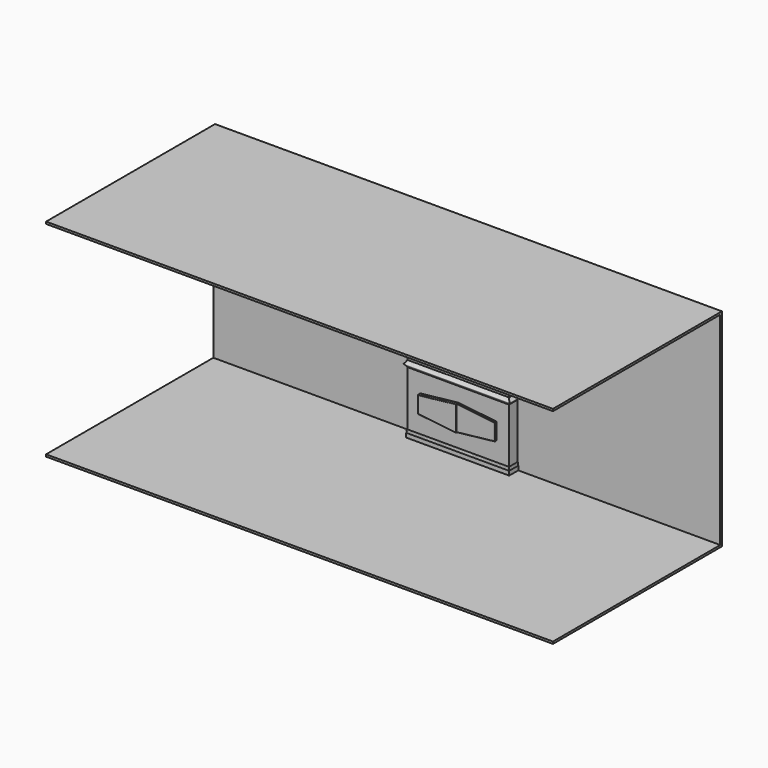
from build123d import *

# Parameters (mm, degrees)
F0_W      = 2438.4
F0_H      = 2438.4
F0_W_2    = 3657.6
F1_DEPTH  = 25.4
F2_W      = 6096
F2_H      = 2540
F3_DEPTH  = 25.4
F4_W      = 6096
F4_H      = 2540
F5_DEPTH  = 25.4
F6_W      = 1219.2
F6_H      = 2133.6
F7_DEPTH  = 127
F8_W      = 762
F8_H      = 762
F9_DEPTH  = 38.1
F15_DEPTH = 190.501
F16_R     = 25.4
F22_DEPTH = 38.1
F23_DEPTH = 25.4
F24_R     = 5.08
F24_2_R   = 5.08
F25_W     = 711.2
F25_H     = 711.2
F26_DEPTH = 6.35


with BuildPart() as f1:
    # F0 (on Front) → F1 (new body)
    with BuildSketch(Plane.XZ):
        with Locations((-1219.2, 1219.2)):
            Rectangle(F0_W, F0_H)
        with Locations((1828.8, 1219.2)):
            Rectangle(F0_W_2, F0_H)
    extrude(amount=-F1_DEPTH)

    # F2 (on face) → F3 (join)
    with BuildSketch(Plane.XY.offset(2438.4)):
        with Locations((609.6, -1244.6)):
            Rectangle(F2_W, F2_H)
    extrude(amount=F3_DEPTH)

    # F4 (on face) → F5 (join)
    with BuildSketch(Plane(origin=(0, 0, 0), x_dir=(1, 0, 0), z_dir=(0, 0, -1))):
        with Locations((609.6, 1244.6)):
            Rectangle(F4_W, F4_H)
    extrude(amount=F5_DEPTH)


with BuildPart() as f7:
    # F6 (on Front) → F7 (new body)
    with BuildSketch(Plane.XZ):
        with Locations((609.6, 1066.8)):
            Rectangle(F6_W, F6_H)
    extrude(amount=F7_DEPTH)


with BuildPart() as f9:
    # F8 (on face) → F9 (new body)
    with BuildSketch(Plane.XZ.offset(127)):
        with Locations((609.6, 1397)):
            Rectangle(F8_W, F8_H)
    extrude(amount=F9_DEPTH)

    # F14 (on face) → F15 (cut, through all)
    with BuildSketch(Plane.XZ.offset(165.1)):
        with BuildLine():
            ThreePointArc((444.5, 1593.85), (442.6401280605, 1598.3401280605), (438.15, 1600.2))
            Line((438.15, 1600.2), (400.05, 1600.2))
            ThreePointArc((400.05, 1600.2), (395.5598719395, 1598.3401280605), (393.7, 1593.85))
            Line((393.7, 1593.85), (393.7, 1200.15))
            ThreePointArc((393.7, 1200.15), (395.5598719395, 1195.6598719395), (400.05, 1193.8))
            Line((400.05, 1193.8), (438.15, 1193.8))
            ThreePointArc((438.15, 1193.8), (442.6401280605, 1195.6598719395), (444.5, 1200.15))
            Line((444.5, 1200.15), (444.5, 1593.85))
        make_face()
        with BuildLine():
            Line((527.05, 1193.8), (565.15, 1193.8))
            ThreePointArc((565.15, 1193.8), (569.6401280605, 1195.6598719395), (571.5, 1200.15))
            Line((571.5, 1200.15), (571.5, 1593.85))
            ThreePointArc((571.5, 1593.85), (569.6401280605, 1598.3401280605), (565.15, 1600.2))
            Line((565.15, 1600.2), (527.05, 1600.2))
            ThreePointArc((527.05, 1600.2), (522.5598719395, 1598.3401280605), (520.7, 1593.85))
            Line((520.7, 1593.85), (520.7, 1200.15))
            ThreePointArc((520.7, 1200.15), (522.5598719395, 1195.6598719395), (527.05, 1193.8))
        make_face()
        with BuildLine():
            Line((654.05, 1193.8), (692.15, 1193.8))
            ThreePointArc((692.15, 1193.8), (696.6401280605, 1195.6598719395), (698.5, 1200.15))
            Line((698.5, 1200.15), (698.5, 1593.85))
            ThreePointArc((698.5, 1593.85), (696.6401280605, 1598.3401280605), (692.15, 1600.2))
            Line((692.15, 1600.2), (654.05, 1600.2))
            ThreePointArc((654.05, 1600.2), (649.5598719395, 1598.3401280605), (647.7, 1593.85))
            Line((647.7, 1593.85), (647.7, 1200.15))
            ThreePointArc((647.7, 1200.15), (649.5598719395, 1195.6598719395), (654.05, 1193.8))
        make_face()
        with BuildLine():
            Line((781.05, 1193.8), (819.15, 1193.8))
            ThreePointArc((819.15, 1193.8), (823.6401280605, 1195.6598719395), (825.5, 1200.15))
            Line((825.5, 1200.15), (825.5, 1593.85))
            ThreePointArc((825.5, 1593.85), (823.6401280605, 1598.3401280605), (819.15, 1600.2))
            Line((819.15, 1600.2), (781.05, 1600.2))
            ThreePointArc((781.05, 1600.2), (776.5598719395, 1598.3401280605), (774.7, 1593.85))
            Line((774.7, 1593.85), (774.7, 1200.15))
            ThreePointArc((774.7, 1200.15), (776.5598719395, 1195.6598719395), (781.05, 1193.8))
        make_face()
    extrude(amount=-F15_DEPTH, mode=Mode.SUBTRACT)

    # F16
    f16_edges = [f9.edges().sort_by_distance(p)[0] for p in [
        (990.6, -165.1, 1397),
        (609.6, -165.1, 1778),
        (228.6, -165.1, 1397),
        (609.6, -165.1, 1016),
    ]]
    fillet(f16_edges, radius=F16_R)

    # F25 (on face) → F26 (join)
    with BuildSketch(Plane.XZ.offset(165.1)):
        with Locations((609.6, 1397)):
            Rectangle(F25_W, F25_H)
        with BuildLine():
            Line((355.6, 1701.8), (863.6, 1701.8))
            ThreePointArc((863.6, 1701.8), (899.5210244843, 1686.9210244843), (914.4, 1651))
            Line((914.4, 1651), (914.4, 1143))
            ThreePointArc((914.4, 1143), (899.5210244843, 1107.0789755157), (863.6, 1092.2))
            Line((863.6, 1092.2), (355.6, 1092.2))
            ThreePointArc((355.6, 1092.2), (319.6789755157, 1107.0789755157), (304.8, 1143))
            Line((304.8, 1143), (304.8, 1651))
            ThreePointArc((304.8, 1651), (319.6789755157, 1686.9210244843), (355.6, 1701.8))
        make_face(mode=Mode.SUBTRACT)
    extrude(amount=F26_DEPTH)


with BuildPart() as f11:
    # F11: sweep along a path in F11_path
    with BuildLine(Plane(origin=(1219.2, -127, 2133.6), x_dir=(0, 1, 0), z_dir=(0, 0, 1))) as f11_path:
        Line((127, 0), (0, 0))
        Line((0, 0), (0, 1219.2))
        Line((0, 1219.2), (127, 1219.2))
    # F10 (on face) → F11 (sweep)
    with BuildSketch(Plane.YZ.offset(1219.2)):
        with BuildLine():
            add(Edge.make_bspline(
                [(-127, 1981.2), (-160.0007931662, 1992.2137728041), (-155.4473179822, 2046.099253464), (-193.9533359526, 2103.7873204418), (-217.0423418283, 2102.3781299591), (-228.6, 2133.6)],
                knots=[0, 0, 0, 0, 0.3678138407, 0.6926670974, 1, 1, 1, 1], degree=3))
            Line((-127, 1981.2), (-127, 2133.6))
            Line((-127, 2133.6), (-228.6, 2133.6))
        make_face()
    sweep(path=f11_path.line, transition=Transition.RIGHT)


with BuildPart() as f18:
    # F18: sweep along a path in F18_path
    with BuildLine(Plane(origin=(0, -127, 0), x_dir=(0, -1, 0), z_dir=(0, 0, -1))) as f18_path:
        Line((-127, 0), (0, 0))
        Line((0, 0), (0, -1219.2))
        Line((0, -1219.2), (-127, -1219.2))
    # F17 (on face) → F18 (sweep)
    with BuildSketch(Plane.YZ.offset(1219.2)):
        with BuildLine():
            Line((-127, 782.5392063567), (-127, 820.6392063567))
            add(Edge.make_bspline(
                [(-127, 820.6392063567), (-134.8272781523, 818.9802669984), (-132.4179834286, 798.1163011268), (-154.2490943357, 788.5070093098), (-153.9875, 782.5392063567)],
                knots=[0, 0, 0, 0, 0.2445921545, 0.5, 0.5, 0.5, 0.5], degree=3))
            Line((-153.9875, 782.5392063567), (-127, 782.5392063567))
        make_face()
        with BuildLine():
            Line((-127, 782.5392063567), (-153.9875, 782.5392063567))
            add(Edge.make_bspline(
                [(-153.9875, 782.5392063567), (-153.7259056643, 776.5714034035), (-130.8705727521, 762.8149174728), (-138.2708600961, 754.0412935956), (-127, 744.4392063567)],
                knots=[0.5, 0.5, 0.5, 0.5, 0.7554078455, 1, 1, 1, 1], degree=3))
            Line((-127, 744.4392063567), (-127, 782.5392063567))
        make_face()
    sweep(path=f18_path.line, transition=Transition.RIGHT)


with BuildPart() as f20:
    # F20: sweep along a path in F20_path
    with BuildLine(Plane(origin=(0, -127, 0), x_dir=(0, -1, 0), z_dir=(0, 0, -1))) as f20_path:
        Line((-127, 0), (0, 0))
        Line((0, 0), (0, -1219.2))
        Line((0, -1219.2), (-127, -1219.2))
    # F19 (on face) → F20 (sweep)
    with BuildSketch(Plane.YZ.offset(1219.2)):
        with BuildLine():
            Line((-136.525, 0), (-127, 0))
            Line((-127, 0), (-127, 85.725))
            add(Edge.make_bspline(
                [(-136.525, 50.8), (-131.9602876902, 54.9347810447), (-132.7376552048, 68.2247962268), (-135.3640973924, 76.7295841133), (-133.2196295261, 85.0994363427), (-127, 85.725)],
                knots=[0, 0, 0, 0, 0.3909258794, 0.6838236064, 1, 1, 1, 1], degree=3))
            Line((-136.525, 50.8), (-136.525, 0))
        make_face()
    sweep(path=f20_path.line, transition=Transition.RIGHT)


with BuildPart() as f22:
    # F21 (on face) → F22 (new body, through all)
    with BuildSketch(Plane.XZ.offset(127)):
        Polygon((609.6, 262.6821031783), (609.6, 567.4821031783), (152.4, 516.6821031783), (152.4, 313.4821031783), align=None)
    extrude(amount=F22_DEPTH)

    # F24
    f24_edges = [f22.edges().sort_by_distance(p)[0] for p in [
        (381, -165.1, 542.082103),
        (381, -165.1, 288.082103),
        (152.4, -165.1, 415.082103),
    ]]
    fillet(f24_edges, radius=F24_R)


with BuildPart() as f23:
    # F21 (on face) → F23 (new body)
    with BuildSketch(Plane.XZ.offset(127)):
        Polygon((1066.8, 516.6821031783), (609.6, 567.4821031783), (609.6, 262.6821031783), (1066.8, 313.4821031783), align=None)
    extrude(amount=F23_DEPTH)

    # F24#2
    f24_2_edges = [f23.edges().sort_by_distance(p)[0] for p in [
        (838.2, -152.4, 542.082103),
        (1066.8, -152.4, 415.082103),
        (838.2, -152.4, 288.082103),
    ]]
    fillet(f24_2_edges, radius=F24_2_R)


solid = Compound([f1.part, f7.part, f9.part, f11.part, f18.part, f20.part, f22.part, f23.part])
